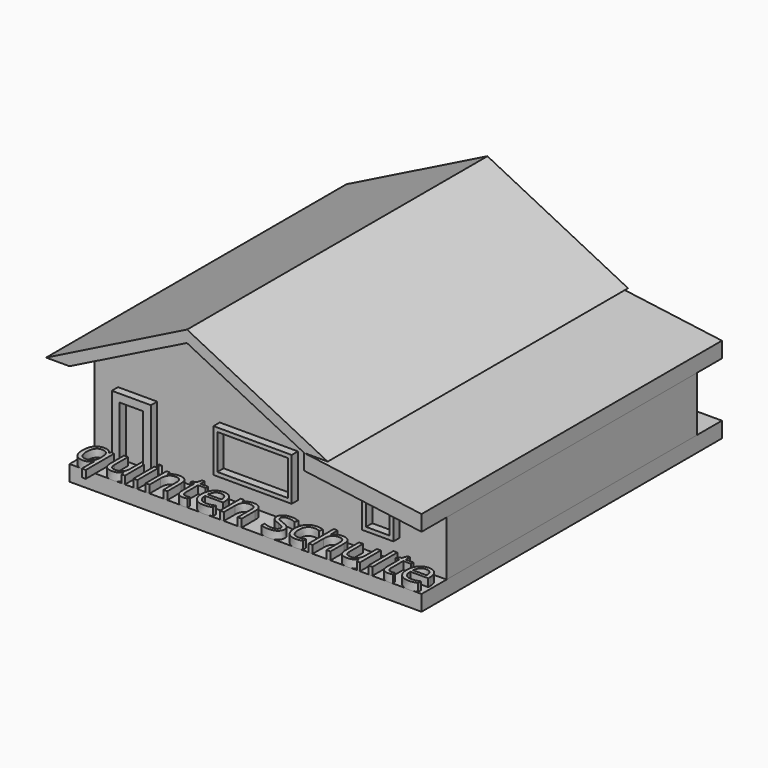
from build123d import *

# Parameters (mm, degrees)
F0_W         = 3048
F0_H         = 1676.4
F0_W_2       = 1219.2
F0_H_2       = 1371.6
F1_DEPTH     = 6096
F0_W_3       = 2743.2
F0_W_4       = 914.4
F0_H_3       = 2133.6
F0_H_4       = 1066.8
F2_DEPTH     = 6400.8
F0_W_5       = 4572
F0_H_5       = 609.6
F3_DEPTH     = 7315.2
F4_TEXT_SIZE = 1894.1889821548
F5_DEPTH     = 304.8


# Not quite as in the source:
# - Text() gives the source's letters only with a copy of the font that has no kerning and outlines rounded to 1/6400 em; it was checked with that copy


with BuildPart() as f1:
    # F0 (on Front) → F1 (new body, symmetric)
    with BuildSketch(Plane.XZ):
        Polygon((4572, 0), (0, 0), (-4572, 0), (-4572, -3352.8), (-3657.6, -3352.8), (-3657.6, -914.4), (-2133.6, -914.4), (-2133.6, -3352.8), (4572, -3352.8), (4572, -609.6), align=None)
        with Locations((1828.8, -1676.4)):
            Rectangle(F0_W, F0_H, mode=Mode.SUBTRACT)
        Polygon((9144, -1219.2), (4572, -609.6), (4572, -3352.8), (9144, -3352.8), align=None)
        with Locations((6705.6, -1828.8)):
            Rectangle(F0_W_2, F0_H_2, mode=Mode.SUBTRACT)
        Polygon((0, 2286), (0, 0), (4572, 0), align=None)
        Polygon((-4572, 0), (0, 0), (0, 2286), align=None)
    extrude(amount=F1_DEPTH, both=True)


with BuildPart() as f1b:
    # F0 (on Front) → F1, piece 2 (new body, symmetric)
    with BuildSketch(Plane.XZ):
        with Locations((1828.8, -1676.4)):
            Rectangle(F0_W_3, F0_H_2)
    extrude(amount=F1_DEPTH, both=True)


with BuildPart() as f1c:
    # F0 (on Front) → F1, piece 3 (new body, symmetric)
    with BuildSketch(Plane.XZ):
        with Locations((-2895.6, -2286)):
            Rectangle(F0_W_4, F0_H_3)
    extrude(amount=F1_DEPTH, both=True)


with BuildPart() as f1d:
    # F0 (on Front) → F1, piece 4 (new body, symmetric)
    with BuildSketch(Plane.XZ):
        with Locations((6705.6, -1828.8)):
            Rectangle(F0_W_4, F0_H_4)
    extrude(amount=F1_DEPTH, both=True)


with BuildPart() as f2:
    # F0 (on Front) → F2 (new body, symmetric)
    with BuildSketch(Plane.XZ):
        Polygon((-3657.6, -914.4), (-3657.6, -3352.8), (-3352.8, -3352.8), (-3352.8, -1219.2), (-2438.4, -1219.2), (-2438.4, -3352.8), (-2133.6, -3352.8), (-2133.6, -914.4), align=None)
    extrude(amount=F2_DEPTH, both=True)


with BuildPart() as f2b:
    # F0 (on Front) → F2, piece 2 (new body, symmetric)
    with BuildSketch(Plane.XZ):
        with Locations((1828.8, -1676.4)):
            Rectangle(F0_W, F0_H)
        with Locations((1828.8, -1676.4)):
            Rectangle(F0_W_3, F0_H_2, mode=Mode.SUBTRACT)
    extrude(amount=F2_DEPTH, both=True)


with BuildPart() as f2c:
    # F0 (on Front) → F2, piece 3 (new body, symmetric)
    with BuildSketch(Plane.XZ):
        with Locations((6705.6, -1828.8)):
            Rectangle(F0_W_2, F0_H_2)
        with Locations((6705.6, -1828.8)):
            Rectangle(F0_W_4, F0_H_4, mode=Mode.SUBTRACT)
    extrude(amount=F2_DEPTH, both=True)


with BuildPart() as f3:
    # F0 (on Front) → F3 (new body, symmetric)
    with BuildSketch(Plane.XZ):
        Polygon((-3657.6, -3352.8), (-4572, -3352.8), (-4572, -3962.4), (4572, -3962.4), (4572, -3352.8), (-2133.6, -3352.8), (-2438.4, -3352.8), (-3352.8, -3352.8), align=None)
        with Locations((6858, -3657.6)):
            Rectangle(F0_W_5, F0_H_5)
    extrude(amount=F3_DEPTH, both=True)


with BuildPart() as f3b:
    # F0 (on Front) → F3, piece 2 (new body, symmetric)
    with BuildSketch(Plane.XZ):
        Polygon((9144, -609.6), (4572, 0), (4572, -609.6), (9144, -1219.2), align=None)
    extrude(amount=F3_DEPTH, both=True)


with BuildPart() as f3c:
    # F0 (on Front) → F3, piece 3 (new body, symmetric)
    with BuildSketch(Plane.XZ):
        Polygon((-5486.4, 0), (-4572, 0), (0, 2286), (4572, 0), (5486.4, 0), (7.7786722791, 2747.0893361396), align=None)
    extrude(amount=F3_DEPTH, both=True)


with BuildPart() as f5:
    # F4 (on face) → F5 (new body)
    with BuildSketch(Plane.XY.offset(-3352.8)):
        with Locations((-4572, -7315.2)):
            Text('quinten schulte', F4_TEXT_SIZE, font='Open Sans', text_align=(TextAlign.LEFT, TextAlign.BOTTOM))
    extrude(amount=F5_DEPTH)


solid = Compound([f1.part, f1b.part, f1c.part, f1d.part, f2.part, f2b.part, f2c.part, f3.part, f3b.part, f3c.part, f5.part])
